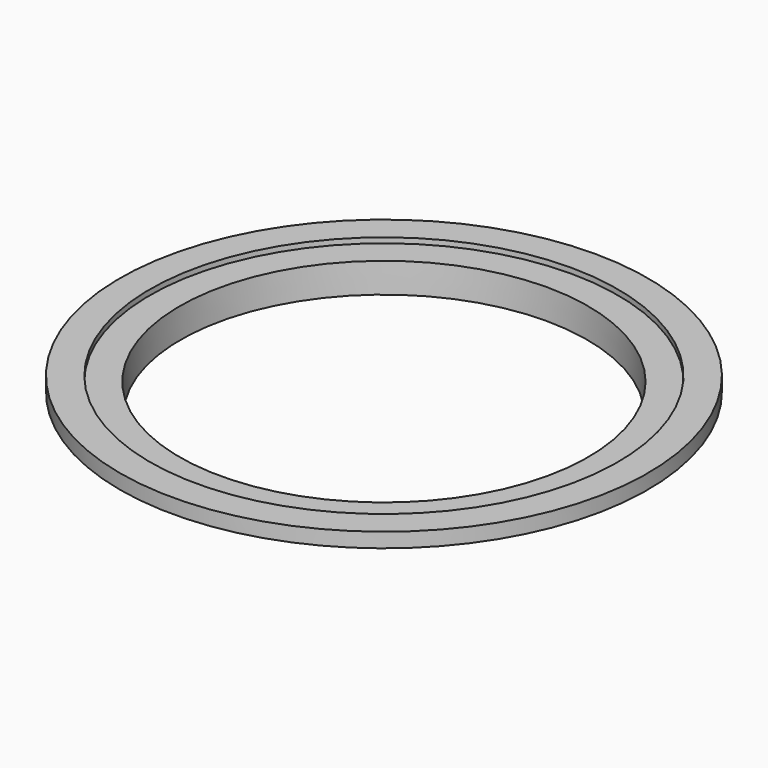
from build123d import *


# Not quite as in the source:
# - a feature of the source that left no trace in its solid (it failed there, or was rolled back) is left out
# - the program builds the solid bodies; features that only make, move or delete a surface that nothing else refers to are left out


with BuildPart() as f1:
    # F0 (on Right) → F1 (revolve)
    with BuildSketch(Plane.YZ):
        Polygon((90.25, 0), (90.25, 5), (80, 5), (80, 3.2), (69.8617464624, 3.2), (69.5125387675, -6.8), (72.5125387675, -6.8), (72.75, 0), align=None)
    revolve(axis=Axis((0, 0, 0), (0, 0, -1)))


solid = f1.part
